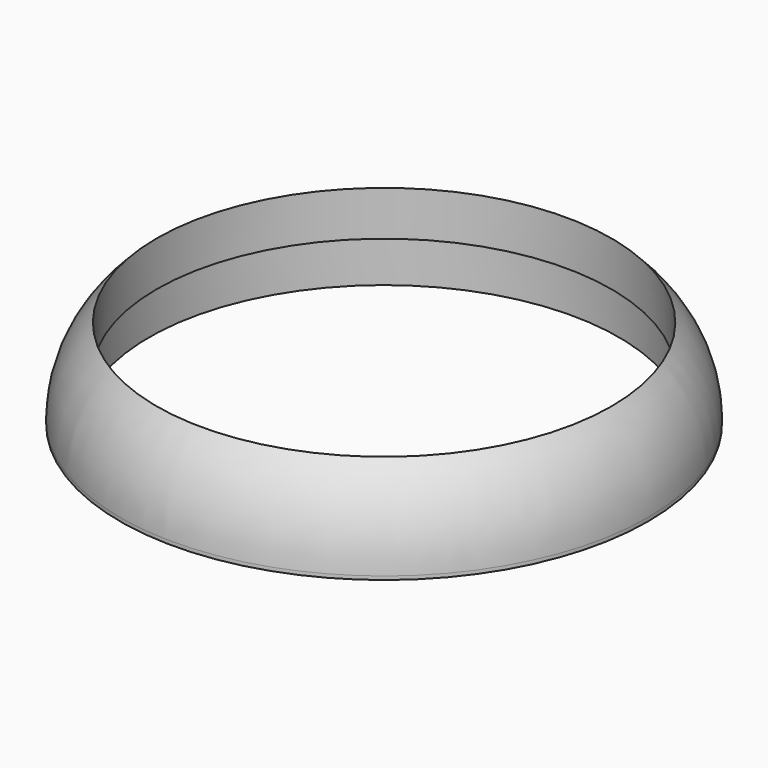
from build123d import *

# Parameters (mm, degrees)
F0_R     = 17.7
F1_DEPTH = 6
F2_R     = 15.75
F3_DEPTH = 3
F4_R     = 15.25
F5_DEPTH = 2
F6_R     = 15.25
F7_DEPTH = 1


# Not quite as in the source:
# - a fillet or chamfer that OpenCascade refuses, or shapes differently, is made with other operations: its cross-section is extruded or revolved along the edge and cut away or added


with BuildPart() as f1:
    # F0 (on Top) → F1 (new body)
    with BuildSketch(Plane.XY):
        Circle(F0_R)
    extrude(amount=F1_DEPTH)

    # F2 (on face) → F3 (cut)
    with BuildSketch(Plane(origin=(0, 0, 0), x_dir=(1, 0, 0), z_dir=(0, 0, -1))):
        Circle(F2_R)
    extrude(amount=-F3_DEPTH, mode=Mode.SUBTRACT)

    # F4 (on face) → F5 (cut)
    with BuildSketch(Plane(origin=(0, 0, 3), x_dir=(1, 0, 0), z_dir=(0, 0, -1))):
        Circle(F4_R)
    extrude(amount=-F5_DEPTH, mode=Mode.SUBTRACT)

    # F6 (on face) → F7 (cut)
    with BuildSketch(Plane.XY.offset(6)):
        Circle(F6_R)
    extrude(amount=-F7_DEPTH, mode=Mode.SUBTRACT)

    # F8: fillet of radius 8 on 1 edges, made by hand

    # F8_s1 → F8_t2 (revolve, cut)
    with BuildSketch(Plane.XZ):
        with BuildLine():
            ThreePointArc((17.7, 0.2382728284), (17.0620649277, 3.3687679969), (15.25, 6))
            Line((15.25, 6), (15.361, 6.1152345434))
            ThreePointArc((15.361, 6.1152345434), (16.475, 6.16), (17.7, 6.16))
            Line((17.7, 6.16), (17.86, 6))
            Line((17.86, 6), (17.86, 0.2382728284))
            Line((17.86, 0.2382728284), (17.7, 0.2382728284))
        make_face()
    revolve(axis=Axis((0, 0, 6), (0, 0, 1)), mode=Mode.SUBTRACT)


solid = f1.part
